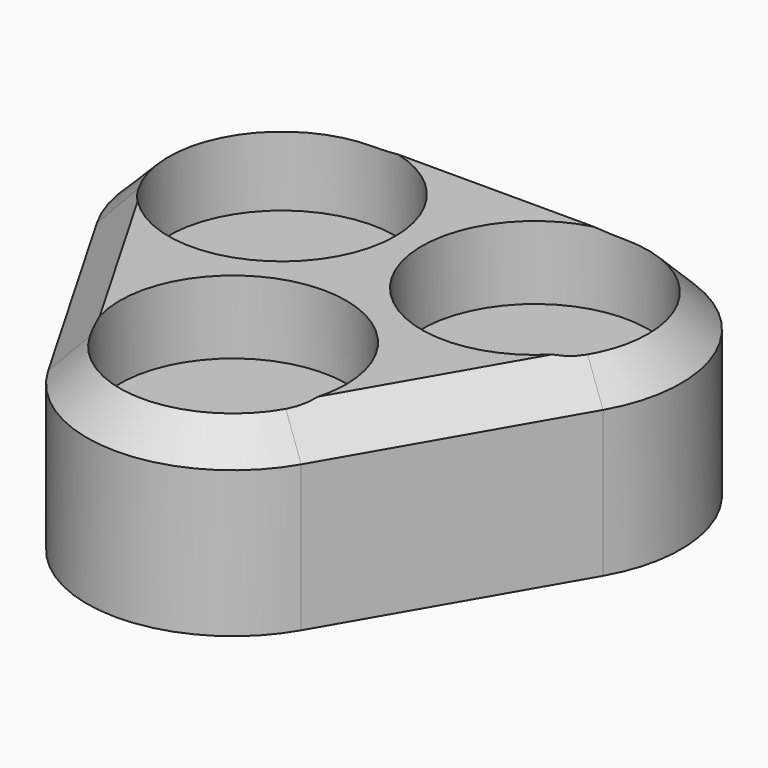
from build123d import *

# Parameters (mm, degrees)
F1_DEPTH     = 25
F2_R         = 15.5
F3_DEPTH     = 10
F4_T1_DEPTH  = 34.6410161514
F4_T3_DEPTH  = 34.6410161514
F4_T5_DEPTH  = 34.6410161514
F4_T8_ANGLE  = 120
F4_T10_ANGLE = 120
F4_T12_ANGLE = 120


# Not quite as in the source:
# - a fillet or chamfer that OpenCascade refuses, or shapes differently, is made with other operations: its cross-section is extruded or revolved along the edge and cut away or added


with BuildPart() as f1:
    # F0 (on Top) → F1 (new body)
    with BuildSketch(Plane.XY):
        with BuildLine():
            Line((17.3205080757, 30), (-17.3205080757, 30))
            ThreePointArc((-17.3205080757, 30), (-34.6410161514, 20), (-34.6410161514, 0))
            Line((-34.6410161514, 0), (-17.3205080757, -30))
            ThreePointArc((-17.3205080757, -30), (0, -40), (17.3205080757, -30))
            Line((17.3205080757, -30), (34.6410161514, 0))
            ThreePointArc((34.6410161514, 0), (34.6410161514, 20), (17.3205080757, 30))
        make_face()
    extrude(amount=F1_DEPTH)

    # F2 (on face) → F3 (cut)
    with BuildSketch(Plane.XY.offset(25)):
        with Locations((-17.3205080757, 10)):
            Circle(F2_R)
        with Locations((0, -20)):
            Circle(F2_R)
        with Locations((17.3205080757, 10)):
            Circle(F2_R)
    extrude(amount=-F3_DEPTH, mode=Mode.SUBTRACT)

    # F4: chamfer of 5 on 1 edges, made by hand

    # F4_s2 → F4_t1 (cut)
    with BuildSketch(Plane(origin=(-8.6602540378, -15, 0), x_dir=(0, 0, 1), z_dir=(0.5, 0.8660254038, 0))):
        Polygon((25, 25), (20, 30), (25, 30), align=None)
    extrude(amount=F4_T1_DEPTH, mode=Mode.SUBTRACT)

    # F4_s4 → F4_t3 (cut)
    with BuildSketch(Plane.YZ.offset(-17.3205080757)):
        Polygon((30, 20), (25, 25), (30, 25), align=None)
    extrude(amount=F4_T3_DEPTH, mode=Mode.SUBTRACT)

    # F4_s6 → F4_t5 (cut)
    with BuildSketch(Plane(origin=(-8.6602540378, 15, 0), x_dir=(0, 0, 1), z_dir=(0.5, -0.8660254038, 0))):
        Polygon((25, 25), (20, 30), (25, 30), align=None)
    extrude(amount=F4_T5_DEPTH, mode=Mode.SUBTRACT)

    # F4_s7 → F4_t8 (revolve, cut)
    with BuildSketch(Plane(origin=(8.6602540378, -15, 0), x_dir=(0, 0, 1), z_dir=(-0.5, 0.8660254038, 0))):
        Polygon((25, -25), (20, -30), (25, -30), align=None)
    revolve(axis=Axis((0, -20, 25), (0, 0, 1)), revolution_arc=F4_T8_ANGLE, mode=Mode.SUBTRACT)

    # F4_s9 → F4_t10 (revolve, cut)
    with BuildSketch(Plane(origin=(8.6602540378, 15, 0), x_dir=(0, 0, 1), z_dir=(-0.5, -0.8660254038, 0))):
        Polygon((20, -30), (25, -25), (25, -30), align=None)
    revolve(axis=Axis((17.3205080757, 10, 25), (0, 0, 1)), revolution_arc=F4_T10_ANGLE, mode=Mode.SUBTRACT)

    # F4_s11 → F4_t12 (revolve, cut)
    with BuildSketch(Plane.YZ.offset(-17.3205080757)):
        Polygon((30, 20), (25, 25), (30, 25), align=None)
    revolve(axis=Axis((-17.3205080757, 10, 25), (0, 0, 1)), revolution_arc=F4_T12_ANGLE, mode=Mode.SUBTRACT)


solid = f1.part
